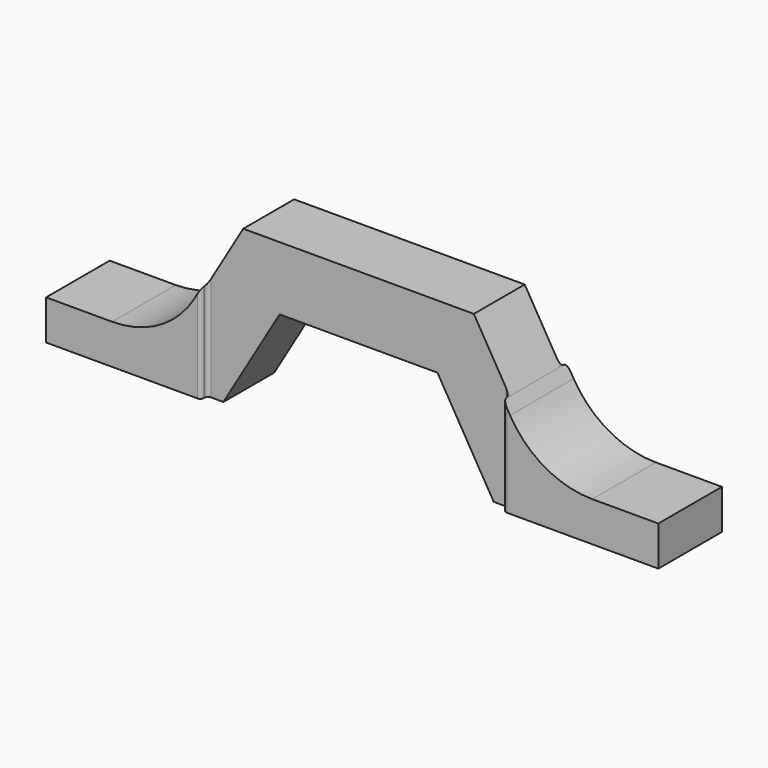
from build123d import *

# Parameters (mm, degrees)
F1_DEPTH     = 25.4
F2_DEPTH     = 31.75
F3_T4_DEPTH  = 86.0090909091
F3_T9_DEPTH  = 86.0090909091
F3_T14_DEPTH = 86.0090909091
F3_T19_DEPTH = 86.0090909091
F3_T21_DEPTH = 93.5090909091


# Not quite as in the source:
# - a fillet or chamfer that OpenCascade refuses, or shapes differently, is made with other operations: its cross-section is extruded or revolved along the edge and cut away or added


with BuildPart() as f1:
    # F0 (on Front) → F1 (new body, symmetric)
    with BuildSketch(Plane.XZ):
        with BuildLine():
            Line((-107.95, -76.2), (-63.0464285714, 0))
            Line((-63.0464285714, 0), (0, 0))
            Line((0, 0), (0, 9.525))
            ThreePointArc((0, 9.525), (8.6950956004, 6.9319779212), (14.5496778315, 0))
            Line((14.5496778315, 0), (63.0464285714, 0))
            Line((63.0464285714, 0), (107.95, -76.2))
            Line((107.95, -76.2), (120.65, -76.2))
            Line((120.65, -76.2), (120.65, 2.3090909091))
            Line((120.65, 2.3090909091), (92.075, 50.8))
            Line((92.075, 50.8), (-92.075, 50.8))
            Line((-92.075, 50.8), (-120.65, 2.3090909091))
            Line((-120.65, 2.3090909091), (-120.65, -76.2))
            Line((-120.65, -76.2), (-107.95, -76.2))
        make_face()
        with BuildLine():
            Line((0, 9.525), (0, 0))
            Line((0, 0), (14.5496778315, 0))
            ThreePointArc((14.5496778315, 0), (8.6950956004, 6.9319779212), (0, 9.525))
        make_face()
    extrude(amount=F1_DEPTH, both=True)

    # F0 (on Front) → F2 (join, symmetric)
    with BuildSketch(Plane.XZ):
        with BuildLine():
            Line((-244.475, -76.2), (-120.65, -76.2))
            Line((-120.65, -76.2), (-120.65, 2.3090909091))
            Line((-120.65, 2.3090909091), (-126.0980906593, -6.9361538462))
            ThreePointArc((-126.0980906593, -6.9361538462), (-153.9415343258, -34.4101274299), (-191.7473214286, -44.45))
            Line((-191.7473214286, -44.45), (-244.475, -44.45))
            Line((-244.475, -44.45), (-244.475, -76.2))
        make_face()
        with BuildLine():
            Line((120.65, 2.3090909091), (120.65, -76.2))
            Line((120.65, -76.2), (244.475, -76.2))
            Line((244.475, -76.2), (244.475, -44.45))
            Line((244.475, -44.45), (191.7473214286, -44.45))
            ThreePointArc((191.7473214286, -44.45), (153.9415343258, -34.4101274299), (126.0980906593, -6.9361538462))
            Line((126.0980906593, -6.9361538462), (120.65, 2.3090909091))
        make_face()
    extrude(amount=F2_DEPTH, both=True)

    # F3: fillet of radius 3 on 8 edges, made by hand


with BuildPart() as f3_tool2:
    # F3_s3 → F3_t4 (new body)
    with BuildSketch(Plane.XY.offset(9.8090909091)):
        with BuildLine():
            ThreePointArc((-120.65, -28.4), (-119.7713203436, -26.2786796564), (-117.65, -25.4))
            Line((-117.65, -25.4), (-120.65, -25.4))
            Line((-120.65, -25.4), (-120.65, -28.4))
        make_face()
    extrude(amount=-F3_T4_DEPTH)

    split(bisect_by=Plane(origin=(-90.5622721893, 0, 53.3670532544), x_dir=(0, 1, 0), z_dir=(0.8615384615, 0, -0.5076923077)), keep=Keep.TOP)


with BuildPart() as f1_1:
    add(f1.part)

    # F3_t1: union F3_tool2
    add(f3_tool2.part)


with BuildPart() as f3_tool7:
    # F3_s8 → F3_t9 (new body)
    with BuildSketch(Plane.XY.offset(9.8090909091)):
        with BuildLine():
            ThreePointArc((-120.65, 28.4), (-119.7713203436, 26.2786796564), (-117.65, 25.4))
            Line((-117.65, 25.4), (-120.65, 25.4))
            Line((-120.65, 25.4), (-120.65, 28.4))
        make_face()
    extrude(amount=-F3_T9_DEPTH)

    split(bisect_by=Plane(origin=(-90.5622721893, 0, 53.3670532544), x_dir=(0, 1, 0), z_dir=(0.8615384615, 0, -0.5076923077)), keep=Keep.TOP)


with BuildPart() as f1_2:
    add(f1_1.part)

    # F3_t6: union F3_tool7
    add(f3_tool7.part)


with BuildPart() as f3_tool12:
    # F3_s13 → F3_t14 (new body)
    with BuildSketch(Plane.XY.offset(-76.2)):
        with BuildLine():
            ThreePointArc((117.65, 25.4), (119.7713203436, 26.2786796564), (120.65, 28.4))
            Line((120.65, 28.4), (120.65, 25.4))
            Line((120.65, 25.4), (117.65, 25.4))
        make_face()
    extrude(amount=F3_T14_DEPTH)

    split(bisect_by=Plane(origin=(90.5622721893, 0, 53.3670532544), x_dir=(0, 1, 0), z_dir=(-0.8615384615, 0, -0.5076923077)), keep=Keep.TOP)


with BuildPart() as f1_3:
    add(f1_2.part)

    # F3_t11: union F3_tool12
    add(f3_tool12.part)


with BuildPart() as f3_tool17:
    # F3_s18 → F3_t19 (new body)
    with BuildSketch(Plane.XY.offset(-76.2)):
        with BuildLine():
            ThreePointArc((117.65, -25.4), (119.7713203436, -26.2786796564), (120.65, -28.4))
            Line((120.65, -28.4), (120.65, -25.4))
            Line((120.65, -25.4), (117.65, -25.4))
        make_face()
    extrude(amount=F3_T19_DEPTH)

    split(bisect_by=Plane(origin=(90.5622721893, 0, 53.3670532544), x_dir=(0, 1, 0), z_dir=(-0.8615384615, 0, -0.5076923077)), keep=Keep.TOP)


with BuildPart() as f1_4:
    add(f1_3.part)

    # F3_t16: union F3_tool17
    add(f3_tool17.part)

    # F3_s22 → F3_t21 (cut)
    with BuildSketch(Plane.XY.offset(-83.7)):
        with BuildLine():
            ThreePointArc((-120.65, -28.75), (-121.5286796564, -30.8713203436), (-123.65, -31.75))
            Line((-123.65, -31.75), (-120.65, -31.75))
            Line((-120.65, -31.75), (-120.65, -28.75))
        make_face()
        with BuildLine():
            ThreePointArc((-123.65, 31.75), (-121.5286796564, 30.8713203436), (-120.65, 28.75))
            Line((-120.65, 28.75), (-120.65, 31.75))
            Line((-120.65, 31.75), (-123.65, 31.75))
        make_face()
        with BuildLine():
            ThreePointArc((120.65, 28.75), (121.5286796564, 30.8713203436), (123.65, 31.75))
            Line((123.65, 31.75), (120.65, 31.75))
            Line((120.65, 31.75), (120.65, 28.75))
        make_face()
        with BuildLine():
            ThreePointArc((123.65, -31.75), (121.5286796564, -30.8713203436), (120.65, -28.75))
            Line((120.65, -28.75), (120.65, -31.75))
            Line((120.65, -31.75), (123.65, -31.75))
        make_face()
    extrude(amount=F3_T21_DEPTH, mode=Mode.SUBTRACT)

    # F0 (on Front) → F4 (revolve, cut)
    with BuildSketch(Plane.XZ):
        with BuildLine():
            Line((0, 9.525), (0, 0))
            Line((0, 0), (14.5496778315, 0))
            ThreePointArc((14.5496778315, 0), (8.6950956004, 6.9319779212), (0, 9.525))
        make_face()
    revolve(axis=Axis((0, 0, 4.7625), (0, 0, -1)), mode=Mode.SUBTRACT)


solid = f1_4.part
